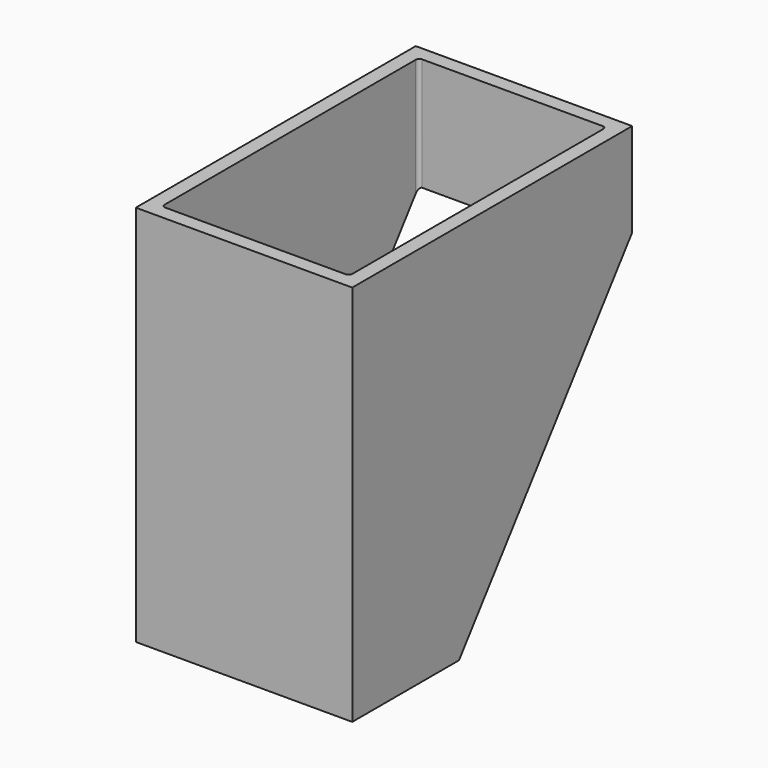
from build123d import *

# Parameters (mm, degrees)
F0_W        = 30
F0_H        = 48.5
F0_W_2      = 26
F0_H_2      = 44.5
F1_DEPTH    = 50
F2_W        = 30
F2_H        = 48.5
F3_DEPTH    = 3
F5_DEPTH    = 30
F6_W        = 4
F6_H        = 14
F7_DEPTH    = 20
F8_R        = 0.5
F9_T1_DEPTH = 14
F9_T3_DEPTH = 19


# Not quite as in the source:
# - a fillet or chamfer that OpenCascade refuses, or shapes differently, is made with other operations: its cross-section is extruded or revolved along the edge and cut away or added


with BuildPart() as f1:
    # F0 (on Top) → F1 (new body)
    with BuildSketch(Plane.XY):
        with Locations((13, -22.25)):
            Rectangle(F0_W, F0_H)
        with Locations((13, -22.25)):
            Rectangle(F0_W_2, F0_H_2, mode=Mode.SUBTRACT)
    extrude(amount=F1_DEPTH)

    # F2 (on face) → F3 (join)
    with BuildSketch(Plane(origin=(0, 0, 0), x_dir=(1, 0, 0), z_dir=(0, 0, -1))):
        with Locations((13, 22.25)):
            Rectangle(F2_W, F2_H)
    extrude(amount=F3_DEPTH)

    # F4 (on face) → F5 (cut)
    with BuildSketch(Plane(origin=(-2, 0, 0), x_dir=(0, -1, 0), z_dir=(-1, 0, 0))):
        Polygon((-2, 37), (-2, -3), (28, -3), align=None)
    extrude(amount=-F5_DEPTH, mode=Mode.SUBTRACT)

    # F6 (on face) → F7 (join)
    with BuildSketch(Plane.XY):
        with Locations((15, -32.75)):
            Rectangle(F6_W, F6_H)
        with Locations((11, -32.75)):
            Rectangle(F6_W, F6_H)
    extrude(amount=F7_DEPTH)

    # F8
    f8_edges = [f1.edges().sort_by_distance(p)[0] for p in [
        (0, -35.125, 0),
        (26, -35.125, 0),
        (0, 0, 42.166667),
        (0, -44.5, 25),
        (26, -44.5, 25),
        (26, 0, 42.166667),
    ]]
    fillet(f8_edges, radius=F8_R)

    # F9: fillet of radius 2 on 4 edges, made by hand

    # F9_s2 → F9_t1 (join)
    with BuildSketch(Plane.XZ.offset(25.75)):
        with BuildLine():
            ThreePointArc((19, 0), (17.5857864376, 0.5857864376), (17, 2))
            Line((17, 2), (17, 0))
            Line((17, 0), (19, 0))
        make_face()
        with BuildLine():
            ThreePointArc((7, 0), (8.4142135624, 0.5857864376), (9, 2))
            Line((9, 2), (9, 0))
            Line((9, 0), (7, 0))
        make_face()
    extrude(amount=F9_T1_DEPTH)

    # F9_s4 → F9_t3 (cut)
    with BuildSketch(Plane.XZ.offset(20.75)):
        with BuildLine():
            ThreePointArc((17, 18), (16.4142135624, 19.4142135624), (15, 20))
            Line((15, 20), (17, 20))
            Line((17, 20), (17, 18))
        make_face()
        with BuildLine():
            ThreePointArc((11, 20), (9.5857864376, 19.4142135624), (9, 18))
            Line((9, 18), (9, 20))
            Line((9, 20), (11, 20))
        make_face()
    extrude(amount=F9_T3_DEPTH, mode=Mode.SUBTRACT)


solid = f1.part
